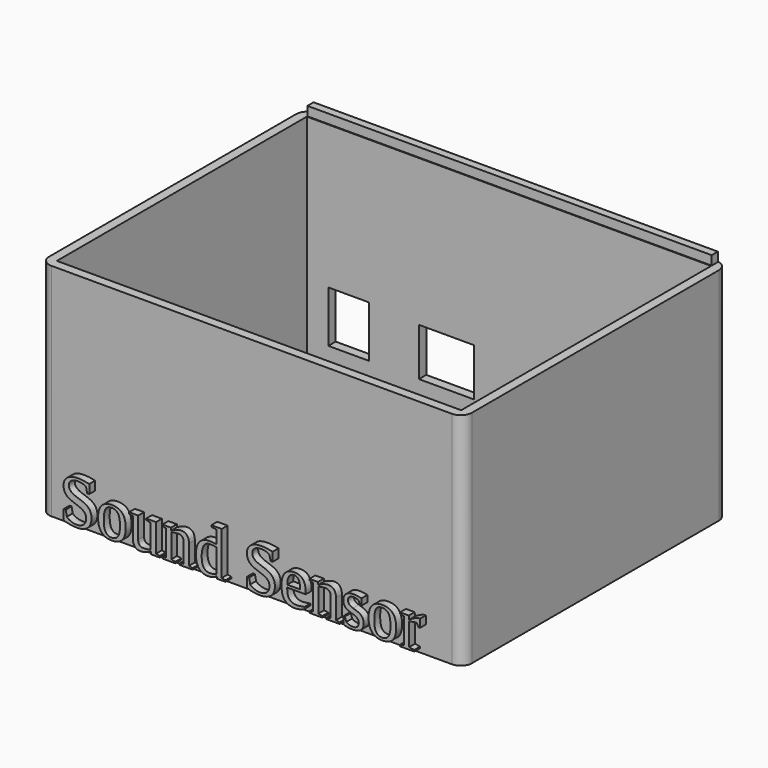
from build123d import *

# Parameters (mm, degrees)
F1_DEPTH     = 60
F2_T         = -2.5
F3_R         = 5
F4_DEPTH     = 2.5
F5_R         = 3
F6_TEXT_SIZE = 17.7792862006
F7_DEPTH     = 2
F8_W         = 2.1
F8_H         = 2.5
F9_DEPTH     = 55


# Not quite as in the source:
# - a feature names something its author has since deleted; it is built from what else it names
# - Text() gives the source's letters only with a copy of the font that has no kerning and outlines rounded to 1/6400 em; it was checked with that copy


with BuildPart() as f1:
    # F0 (on Top) → F1 (new body)
    with BuildSketch(Plane.XY):
        Polygon((57.5, 43.8723909892), (-57.5, 43.8723909892), (-57.5, -46.1276090108), (57.5, -46.1276090108), (57.5, 29.3404459953), align=None)
    extrude(amount=F1_DEPTH)

    # F2
    f2_openings = [f1.faces().sort_by_distance(p)[0] for p in [
        (0, -1.127609, 60),
    ]]
    offset(amount=F2_T, openings=f2_openings)

    # F3 (on face) → F4 (cut)
    with BuildSketch(Plane(origin=(0, 43.8723909892, 0), x_dir=(-1, 0, 0), z_dir=(0, 1, 0))):
        Polygon((38.141977042, 21), (38.141977042, 17.9649144411), (38.141977042, 7), (49.141977042, 7), (49.141977042, 21), align=None)
        Polygon((24.5, 20.0491060615), (9.5, 20.0491060615), (9.5, 7.0491060615), (24.5, 7.0491060615), (24.5, 17.9649144411), align=None)
        with Locations((-39.2560008893, 15.0449005464)):
            Circle(F3_R)
    extrude(amount=-F4_DEPTH, mode=Mode.SUBTRACT)

    # F5
    f5_edges = [f1.edges().sort_by_distance(p)[0] for p in [
        (57.5, -46.127609, 30),
        (-57.5, -46.127609, 30),
        (-57.5, 43.872391, 30),
        (57.5, 43.872391, 30),
    ]]
    fillet(f5_edges, radius=F5_R)

    # F6 (on face) → F7 (join)
    with BuildSketch(Plane.XZ.offset(46.1276090108)):
        with Locations((-50.7647069171, 1.0372239631)):
            Text('Sound Sensor', F6_TEXT_SIZE, font='Tinos', text_align=(TextAlign.LEFT, TextAlign.BOTTOM))
    extrude(amount=F7_DEPTH)


with BuildPart() as f9:
    # F8 (on Right) → F9 (new body, symmetric)
    with BuildSketch(Plane.YZ):
        with Locations((42.6223909892, 61.2513546646)):
            Rectangle(F8_W, F8_H)
    extrude(amount=F9_DEPTH, both=True)


solid = Compound([f1.part, f9.part])
